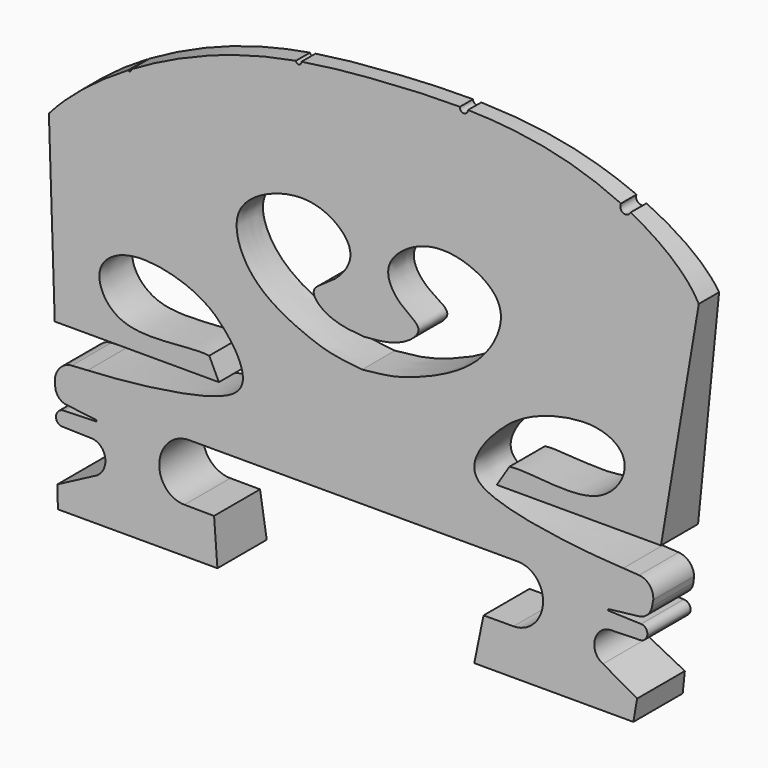
from build123d import *

# Parameters (mm, degrees)
F1_DEPTH     = 4.5
F2_W         = 3.3498070063
F2_H         = 7.5584488809
F2_W_2       = 3.3
F3_DEPTH     = 30
F4_TEXT_SIZE = 3.6633987394
F5_DEPTH     = 0.4


# Not quite as in the source:
# - Text() gives the source's letters only with a copy of the font that has no kerning and outlines rounded to 1/6400 em; it was checked with that copy


with BuildPart() as f1:
    # F0 (on Front) → F1 (new body)
    with BuildSketch(Plane.XZ):
        with BuildLine():
            add(Edge.make_bspline(
                [(-23.5363684416, 23.6552466143), (-22.1809019264, 25.260476146), (-20.2464861976, 26.7563188513), (-18.0861577118, 28.0338079465)],
                knots=[0, 0, 0, 0, 0.1369727751, 0.1369727751, 0.1369727751, 0.1369727751], degree=3))
            Line((-23.5363684416, 23.6552466143), (-22.1226862941, 11.2478661411))
            Line((-22.1226862941, 11.2478661411), (-10.1413011026, 11.2478661411))
            Line((-10.1413011026, 11.2478661411), (-10.9565548074, 12.6261684135))
            add(Edge.make_bspline(
                [(-10.9565548074, 12.6261684135), (-12.4506641968, 12.8114152239), (-17.5784573788, 11.593366016), (-19.9542721652, 15.5722727054), (-16.9274393882, 17.4706918876), (-12.0661208387, 16.3349092226), (-9.9290292696, 14.597388434), (-8.3579108066, 12.6419633785), (-8.3347769443, 9.808542041), (-17.9377850145, 9.0874703601), (-19.545920327, 9.0387157187)],
                knots=[0, 0, 0, 0, 0.1580093991, 0.2698140689, 0.3715152315, 0.5099826839, 0.6153121531, 0.7112759384, 0.7964222327, 1, 1, 1, 1], degree=3))
            Line((-19.545920327, 9.0387157187), (-20.7062717527, 8.9688422158))
            ThreePointArc((-20.7062717527, 8.9688422158), (-21.4957271459, 8.6062784025), (-21.8336324124, 7.8059582369))
            Line((-21.8336324124, 7.8059582369), (-21.7818409617, 7.3668043929))
            ThreePointArc((-21.7818409617, 7.3668043929), (-21.4931945785, 6.7741946047), (-20.8984533479, 6.4899658866))
            Line((-20.8984533479, 6.4899658866), (-18.7077316523, 6.2481180034))
            ThreePointArc((-18.7077316523, 6.2481180034), (-18.6632562021, 6.196469421), (-18.7116228626, 6.1484453865))
            Line((-18.7116228626, 6.1484453865), (-21.0796462954, 6.0728536862))
            ThreePointArc((-21.0796462954, 6.0728536862), (-21.4528495096, 5.9055988754), (-21.5763725918, 5.5157311299))
            Line((-21.5763725918, 5.5157311299), (-21.5706603362, 5.4660585002))
            ThreePointArc((-21.5706603362, 5.4660585002), (-21.3986794627, 5.1939304371), (-21.0964645838, 5.0830373776))
            Line((-21.0964645838, 5.0830373776), (-18.9640834262, 5.0320074941))
            ThreePointArc((-18.9640834262, 5.0320074941), (-17.8633354114, 4.092801096), (-18.5576565569, 2.8232842598))
            Line((-18.5576565569, 2.8232842598), (-21.1583454526, 1.4914511856))
            Line((-21.1583454526, 1.4914511856), (-20.9984287212, 0))
            Line((-20.9984287212, 0), (-9.3567522388, 0))
            Line((-9.3567522388, 0), (-9.8450887185, 3.0820087418))
            Line((-9.8450887185, 3.0820087418), (-12.0103669021, 3.0932325061))
            ThreePointArc((-12.0103669021, 3.0932325061), (-13.9999932829, 5.0983891062), (-12, 7.0932056377))
            Line((-12, 7.0932056377), (0, 7.0932056377))
            Line((0, 7.0932056377), (12, 7.0932056377))
            ThreePointArc((12, 7.0932056377), (13.9999969278, 5.0967111581), (12.0070110301, 3.0932179264))
            Line((12.0070110301, 3.0932179264), (9.8222481397, 3.0855591602))
            Line((9.8222481397, 3.0855591602), (9.3886010798, 0))
            Line((9.3886010798, 0), (21.0015712788, -0.000333604))
            Line((21.0015712788, -0.000333604), (21.1583454526, 1.4914511856))
            Line((21.1583454526, 1.4914511856), (18.5576565569, 2.8232842598))
            ThreePointArc((18.5576565569, 2.8232842598), (17.8633354114, 4.092801096), (18.9640834262, 5.0320074941))
            Line((18.9640834262, 5.0320074941), (21.0964645838, 5.0830373776))
            ThreePointArc((21.0964645838, 5.0830373776), (21.3986794627, 5.1939304371), (21.5706603362, 5.4660585002))
            Line((21.5706603362, 5.4660585002), (21.5763725918, 5.5157311299))
            ThreePointArc((21.5763725918, 5.5157311299), (21.4528495096, 5.9055988754), (21.0796462954, 6.0728536862))
            Line((21.0796462954, 6.0728536862), (18.7116228626, 6.1484453865))
            ThreePointArc((18.7116228626, 6.1484453865), (18.6632562021, 6.196469421), (18.7077316523, 6.2481180034))
            Line((18.7077316523, 6.2481180034), (20.8984533479, 6.4899658866))
            ThreePointArc((20.8984533479, 6.4899658866), (21.4931945785, 6.7741946047), (21.7818409617, 7.3668043929))
            Line((21.7818409617, 7.3668043929), (21.8336324124, 7.8059582369))
            ThreePointArc((21.8336324124, 7.8059582369), (21.4957271459, 8.6062784025), (20.7062717527, 8.9688422158))
            Line((20.7062717527, 8.9688422158), (19.545920327, 9.0387157187))
            add(Edge.make_bspline(
                [(10.9565548074, 12.6261684135), (12.4506641968, 12.8114152239), (17.5784573788, 11.593366016), (19.9542721652, 15.5722727054), (16.9274393882, 17.4706918876), (12.0661208387, 16.3349092226), (9.9290292696, 14.597388434), (8.3579108066, 12.6419633785), (8.3347769443, 9.808542041), (17.9377850145, 9.0874703601), (19.545920327, 9.0387157187)],
                knots=[0, 0, 0, 0, 0.1580093991, 0.2698140689, 0.3715152315, 0.5099826839, 0.6153121531, 0.7112759384, 0.7964222327, 1, 1, 1, 1], degree=3))
            Line((10.9565548074, 12.6261684135), (10.1413011026, 11.2478661411))
            Line((10.1413011026, 11.2478661411), (22.1226862941, 11.2478661411))
            Line((22.1226862941, 11.2478661411), (23.6598201241, 26.6479611198))
            add(Edge.make_bspline(
                [(18.3638422533, 30.6360920918), (20.7414594365, 29.525659305), (22.7102987642, 28.1182143601), (23.6598201241, 26.6479611198)],
                knots=[0.851348028, 0.851348028, 0.851348028, 0.851348028, 1, 1, 1, 1], degree=3))
            ThreePointArc((18.3638422533, 30.6360920918), (17.8368362551, 30.4370722143), (17.6334494669, 30.962408343))
            add(Edge.make_bspline(
                [(6.299949222, 33.1952163198), (8.8406655698, 33.1403760478), (12.7089048862, 32.7453965852), (16.4623871501, 31.4626658371), (17.6334494669, 30.962408343)],
                knots=[0.6233705909, 0.6233705909, 0.6233705909, 0.6233705909, 0.7654288362, 0.8363726665, 0.8363726665, 0.8363726665, 0.8363726665], degree=3))
            ThreePointArc((6.299949222, 33.1952163198), (5.9954147324, 32.9007708022), (5.7000222178, 33.2043868105))
            add(Edge.make_bspline(
                [(-5.8025069017, 32.3939596743), (-3.9020740666, 32.693179971), (-0.2174126257, 33.0225352164), (3.7593850718, 33.2220932827), (5.7000222178, 33.2043868105)],
                knots=[0.3860705679, 0.3860705679, 0.3860705679, 0.3860705679, 0.5033806167, 0.6121750006, 0.6121750006, 0.6121750006, 0.6121750006], degree=3))
            ThreePointArc((-5.8025069017, 32.3939596743), (-5.8006277105, 32.3782258626), (-5.8, 32.3623926643))
            ThreePointArc((-5.8, 32.3623926643), (-5.9836956637, 32.1630583506), (-6.1973416862, 32.3298925274))
            add(Edge.make_bspline(
                [(-17.9136809927, 28.135058526), (-16.0575985182, 29.2167312118), (-11.9733823838, 31.0824601466), (-8.1447664633, 32.0043795548), (-6.1973416862, 32.3298925274)],
                knots=[0.1406080449, 0.1406080449, 0.1406080449, 0.1406080449, 0.2576542794, 0.3779435559, 0.3779435559, 0.3779435559, 0.3779435559], degree=3))
            ThreePointArc((-17.9136809927, 28.135058526), (-17.903480829, 28.1107249593), (-17.9, 28.0845706167))
            ThreePointArc((-17.9, 28.0845706167), (-17.9736919327, 27.9880932329), (-18.0861577118, 28.0338079465))
        make_face()
        with BuildLine():
            add(Edge.make_bspline(
                [(0, 15.1957957089), (2.0903856573, 15.3791947525), (3.6702107386, 15.777829192), (8.5046642167, 17.7997724532), (10.4334916547, 22.0389484407), (7.17305578, 24.1425953549), (3.6327140381, 24.4256207343), (0.659762582, 22.1035580099), (2.2932652276, 19.8200812112), (4.4103600725, 18.9883550435), (2.6764111625, 17.4313099969), (0.8823938701, 17.2681713059), (0, 17.2159889728)],
                knots=[0, 0, 0, 0, 0.1171327199, 0.2437561037, 0.355967299, 0.4582118124, 0.5680705646, 0.6675254018, 0.7551120606, 0.8310829496, 0.9031037961, 1, 1, 1, 1], degree=3))
            add(Edge.make_bspline(
                [(0, 15.1957957089), (-2.0903856573, 15.3791947525), (-3.6702107386, 15.777829192), (-8.5046642167, 17.7997724532), (-10.4334916547, 22.0389484407), (-7.17305578, 24.1425953549), (-3.6327140381, 24.4256207343), (-0.659762582, 22.1035580099), (-2.2932652276, 19.8200812112), (-4.4103600725, 18.9883550435), (-2.6764111625, 17.4313099969), (-0.8823938701, 17.2681713059), (0, 17.2159889728)],
                knots=[0, 0, 0, 0, 0.1171327199, 0.2437561037, 0.355967299, 0.4582118124, 0.5680705646, 0.6675254018, 0.7551120606, 0.8310829496, 0.9031037961, 1, 1, 1, 1], degree=3))
        make_face(mode=Mode.SUBTRACT)
    extrude(amount=F1_DEPTH)

    # F2 (on Right) → F3 (cut, symmetric)
    with BuildSketch(Plane.YZ):
        Polygon((-4.5, 0), (-4.5, 33.213060528), (-7.8498070063, 33.213060528), (-9.0029938146, 0), align=None)
        Polygon((-4.5, 0), (-1.2, 33.213060528), (-4.5, 33.213060528), align=None)
        with Locations((-6.1749035031, 36.9922849685)):
            Rectangle(F2_W, F2_H)
        with Locations((-2.85, 36.9922849685)):
            Rectangle(F2_W_2, F2_H)
    extrude(amount=F3_DEPTH, both=True, mode=Mode.SUBTRACT)

    # F4 (on face) → F5 (cut)
    with BuildSketch(Plane(origin=(0, 0, 0), x_dir=(-1, 0, 0), z_dir=(0, 1, 0))):
        with Locations((-6.1517595313, 10.8835203573)):
            Text('justnth', F4_TEXT_SIZE, font='Open Sans', text_align=(TextAlign.LEFT, TextAlign.BOTTOM))
    extrude(amount=-F5_DEPTH, mode=Mode.SUBTRACT)


solid = f1.part
